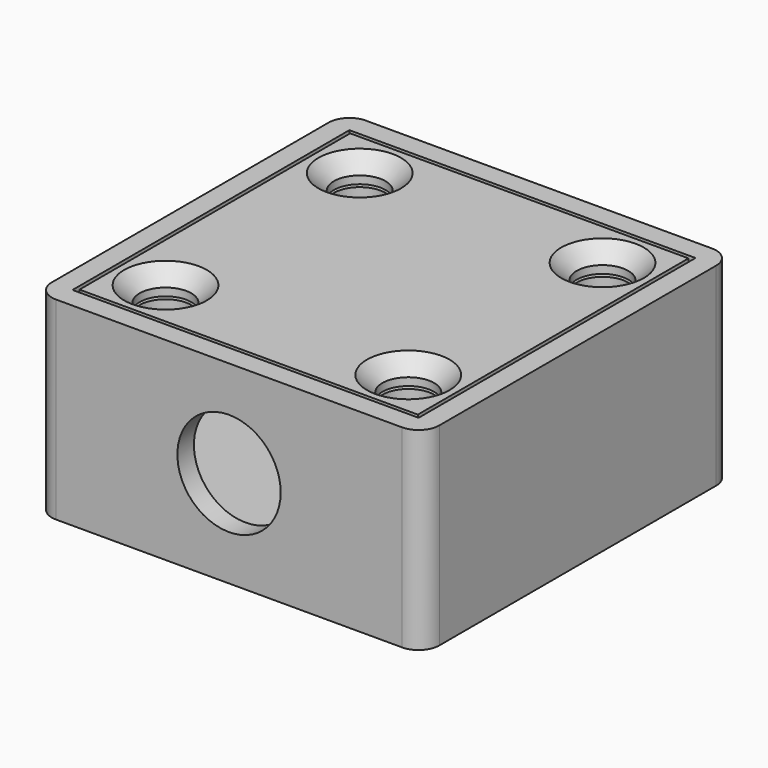
from build123d import *

# Parameters (mm, degrees)
F0_W         = 30
F0_H         = 30
F1_DEPTH     = 15
F2_T         = -1.6
F4_W         = 8
F4_H         = 8
F4_R         = 2
F5_DEPTH     = 10
F6_T4_DEPTH  = 28.5734639037
F6_T9_DEPTH  = 28.5734639037
F6_T14_DEPTH = 28.5734639037
F6_T19_DEPTH = 28.5734639037
F7_R         = 4
F8_DEPTH     = 1.6
F9_W         = 26.2
F9_H         = 26.2
F9_R         = 2
F10_DEPTH    = 1.8
F11_SIZE     = 1.2
F12_R        = 1.6


# Not quite as in the source:
# - a fillet or chamfer that OpenCascade refuses, or shapes differently, is made with other operations: its cross-section is extruded or revolved along the edge and cut away or added


with BuildPart() as f1:
    # F0 (on Top) → F1 (new body)
    with BuildSketch(Plane.XY):
        with Locations((-15, 15)):
            Rectangle(F0_W, F0_H)
    extrude(amount=F1_DEPTH)

    # F2
    f2_openings = [f1.faces().sort_by_distance(p)[0] for p in [
        (-15, 15, 15),
    ]]
    offset(amount=F2_T, openings=f2_openings)

    # F4 (on offset) → F5 (join)
    with BuildSketch(Plane.XY.offset(13)):
        with Locations((-24.4, 24.4)):
            Rectangle(F4_W, F4_H)
        with Locations((-24.4, 24.4)):
            Circle(F4_R, mode=Mode.SUBTRACT)
        with Locations((-5.6, 24.4)):
            Rectangle(F4_W, F4_H)
        with Locations((-5.6, 24.4)):
            Circle(F4_R, mode=Mode.SUBTRACT)
        with Locations((-5.6, 5.6)):
            Rectangle(F4_W, F4_H)
        with Locations((-5.6, 5.6)):
            Circle(F4_R, mode=Mode.SUBTRACT)
        with Locations((-24.4, 5.6)):
            Rectangle(F4_W, F4_H)
        with Locations((-24.4, 5.6)):
            Circle(F4_R, mode=Mode.SUBTRACT)
    extrude(amount=-F5_DEPTH)

    # F6: chamfer of 8 on 4 edges, made by hand


with BuildPart() as f6_tool2:
    # F6_s3 → F6_t4 (new body)
    with BuildSketch(Plane.XZ.offset(0.1734639037)):
        Polygon((-28.4, 3), (-20.4, 11), (-20.4, 3), align=None)
    extrude(amount=-F6_T4_DEPTH)

    split(bisect_by=Plane.XZ.offset(-1.6), keep=Keep.BOTTOM)


with BuildPart() as f1_1:
    add(f1.part)

    # F6_t1: cut F6_tool2
    add(f6_tool2.part, mode=Mode.SUBTRACT)


with BuildPart() as f6_tool7:
    # F6_s8 → F6_t9 (new body)
    with BuildSketch(Plane.XZ.offset(-28.4)):
        Polygon((-9.6, 11), (-1.6, 3), (-9.6, 3), align=None)
    extrude(amount=F6_T9_DEPTH)

    split(bisect_by=Plane.XZ.offset(-1.6), keep=Keep.BOTTOM)


with BuildPart() as f1_2:
    add(f1_1.part)

    # F6_t6: cut F6_tool7
    add(f6_tool7.part, mode=Mode.SUBTRACT)


with BuildPart() as f6_tool12:
    # F6_s13 → F6_t14 (new body)
    with BuildSketch(Plane.XZ.offset(-30.1734639037)):
        Polygon((-1.6, 3), (-9.6, 11), (-9.6, 3), align=None)
    extrude(amount=F6_T14_DEPTH)

    split(bisect_by=Plane.XZ.offset(-28.4), keep=Keep.TOP)


with BuildPart() as f1_3:
    add(f1_2.part)

    # F6_t11: cut F6_tool12
    add(f6_tool12.part, mode=Mode.SUBTRACT)


with BuildPart() as f6_tool17:
    # F6_s18 → F6_t19 (new body)
    with BuildSketch(Plane.XZ.offset(-1.6)):
        Polygon((-20.4, 11), (-28.4, 3), (-20.4, 3), align=None)
    extrude(amount=-F6_T19_DEPTH)

    split(bisect_by=Plane.XZ.offset(-28.4), keep=Keep.TOP)


with BuildPart() as f1_4:
    add(f1_3.part)

    # F6_t16: cut F6_tool17
    add(f6_tool17.part, mode=Mode.SUBTRACT)

    # F7 (on face) → F8 (cut, through all)
    with BuildSketch(Plane.XZ):
        with Locations((-15, 7.5)):
            Circle(F7_R)
    extrude(amount=-F8_DEPTH, mode=Mode.SUBTRACT)

    # F12
    f12_edges = [f1_4.edges().sort_by_distance(p)[0] for p in [
        (0, 30, 7.5),
        (-30, 30, 7.5),
        (-30, 0, 7.5),
        (0, 0, 7.5),
    ]]
    fillet(f12_edges, radius=F12_R)


with BuildPart() as f10:
    # F9 (on face) → F10 (new body)
    with BuildSketch(Plane.XY.offset(15)):
        with Locations((-15, 15)):
            Rectangle(F9_W, F9_H)
        with Locations((-24.4, 5.6)):
            Circle(F9_R, mode=Mode.SUBTRACT)
        with Locations((-5.6, 5.6)):
            Circle(F9_R, mode=Mode.SUBTRACT)
        with Locations((-24.4, 24.4)):
            Circle(F9_R, mode=Mode.SUBTRACT)
        with Locations((-5.6, 24.4)):
            Circle(F9_R, mode=Mode.SUBTRACT)
    extrude(amount=-F10_DEPTH)

    # F11
    f11_edges = [f10.edges().sort_by_distance(p)[0] for p in [
        (-7.6, 24.4, 15),
        (-7.6, 5.6, 15),
        (-26.4, 5.6, 15),
        (-26.4, 24.4, 15),
    ]]
    chamfer(f11_edges, length=F11_SIZE)


solid = Compound([f1_4.part, f10.part])
